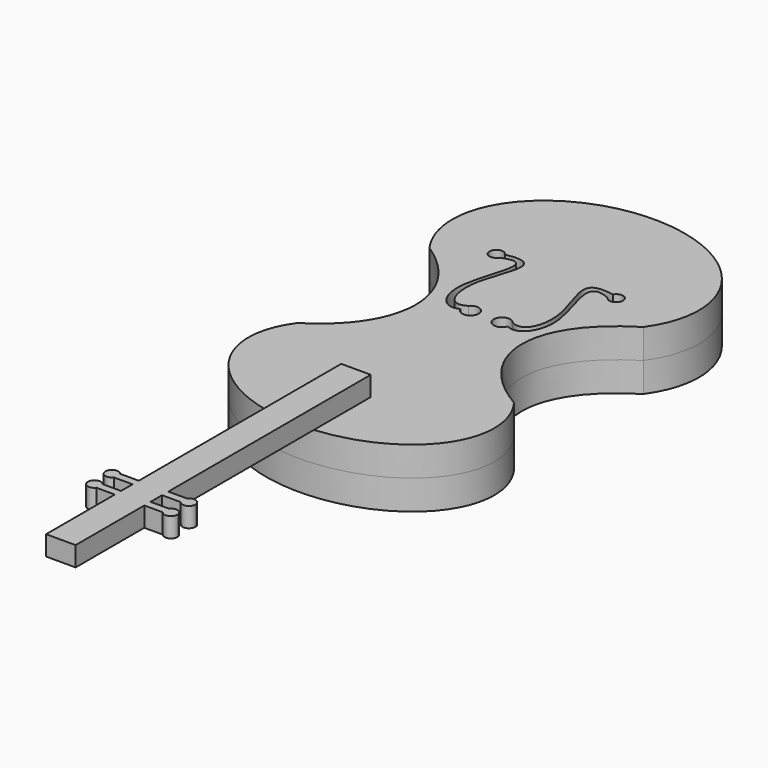
from build123d import *

# Parameters (mm, degrees)
F1_DEPTH = 6
F3_DEPTH = 6
F5_DEPTH = 4
F6_DEPTH = 4


with BuildPart() as f1:
    # F0 (on Top) → F1 (new body)
    with BuildSketch(Plane.XY):
        with BuildLine():
            add(Edge.make_bspline(
                [(-21.7444925397, 18.2306537), (-7.7311441191, 9.1459075591), (-7.7311441191, -6.1719642271), (-21.9778431403, -14.9497014101)],
                knots=[0, 0, 0, 0, 33.1811756533, 33.1811756533, 33.1811756533, 33.1811756533], degree=3))
            add(Edge.make_bspline(
                [(-21.9778431403, -14.9497014101), (-41.9382653472, -42.22478633), (0, -42.22478633), (41.9382653472, -42.22478633), (21.9778431403, -14.9497014101)],
                knots=[2.6455513247, 2.6455513247, 2.6455513247, 4.7123889804, 4.7123889804, 6.779226636, 6.779226636, 6.779226636], degree=2, weights=[1, 0.5118848843, 1, 0.5118848843, 1]))
            add(Edge.make_bspline(
                [(21.7444925397, 18.2306537), (6.4069386012, 8.8349419962), (6.5856454991, -5.9186217795), (21.9778431403, -14.9497014101)],
                knots=[0, 0, 0, 0, 33.1811756533, 33.1811756533, 33.1811756533, 33.1811756533], degree=3))
            add(Edge.make_bspline(
                [(21.7444925397, 18.2306537), (43.2497024841, 48.1910994303), (0, 48.1910994303), (-43.2497024841, 48.1910994303), (-21.7444925397, 18.2306537)],
                knots=[5.7627778356, 5.7627778356, 5.7627778356, 7.853981634, 7.853981634, 9.9451854323, 9.9451854323, 9.9451854323], degree=2, weights=[1, 0.5013812381, 1, 0.5013812381, 1]))
        make_face()
    extrude(amount=F1_DEPTH)

    # F2 (on face) → F3 (join)
    with BuildSketch(Plane.XY.offset(6)):
        with BuildLine():
            add(Edge.make_bspline(
                [(21.7444925397, 18.2306537), (43.2497024841, 48.1910994303), (0, 48.1910994303), (-43.2497024841, 48.1910994303), (-21.7444925397, 18.2306537)],
                knots=[5.7627778356, 5.7627778356, 5.7627778356, 7.853981634, 7.853981634, 9.9451854323, 9.9451854323, 9.9451854323], degree=2, weights=[1, 0.5013812381, 1, 0.5013812381, 1]))
            add(Edge.make_bspline(
                [(-21.7444925397, 18.2306537), (-7.7311441191, 9.1459075591), (-7.7311441191, -6.1719642271), (-21.9778431403, -14.9497014101)],
                knots=[0, 0, 0, 0, 33.1811756533, 33.1811756533, 33.1811756533, 33.1811756533], degree=3))
            add(Edge.make_bspline(
                [(-21.9778431403, -14.9497014101), (-41.9382653472, -42.22478633), (0, -42.22478633), (41.9382653472, -42.22478633), (21.9778431403, -14.9497014101)],
                knots=[2.6455513247, 2.6455513247, 2.6455513247, 4.7123889804, 4.7123889804, 6.779226636, 6.779226636, 6.779226636], degree=2, weights=[1, 0.5118848843, 1, 0.5118848843, 1]))
            add(Edge.make_bspline(
                [(21.7444925397, 18.2306537), (6.4069386012, 8.8349419962), (6.5856454991, -5.9186217795), (21.9778431403, -14.9497014101)],
                knots=[0, 0, 0, 0, 33.1811756533, 33.1811756533, 33.1811756533, 33.1811756533], degree=3))
        make_face()
        with BuildLine():
            add(Edge.make_bspline(
                [(-10.9988739486, 22.5408715923), (-4.1913907555, 25.4376747874), (-13.3990144667, 10.0652438331), (-7.4404065422, 3.5960169038), (-4.885258902, 4.8904192687)],
                knots=[0, 0, 0, 0, 0.5395747944, 1, 1, 1, 1], degree=3))
            ThreePointArc((-10.9988739486, 22.5408715923), (-13.5682932315, 23.2902762166), (-10.9684085473, 23.9259824157))
            add(Edge.make_bspline(
                [(-10.9684085473, 23.9259824157), (-3.068382332, 25.4376747874), (-11.2785667863, 14.0586412607), (-7.7607951045, 4.559221291), (-4.5054177754, 6.5329330973)],
                knots=[0, 0, 0, 0, 0.5227502867, 1, 1, 1, 1], degree=3))
            ThreePointArc((-4.5054177754, 6.5329330973), (-2.6347231367, 7.0482026203), (-1.5180834207, 5.4613450788))
            ThreePointArc((-1.5180834207, 5.4613450788), (-2.9141698346, 3.8005738661), (-4.7901909683, 4.8904192687))
            Line((-4.7901909683, 4.8904192687), (-4.885258902, 4.8904192687))
        make_face(mode=Mode.SUBTRACT)
        with BuildLine():
            ThreePointArc((13.568628233, 23.2598108154), (12.5564550452, 21.9255965626), (10.9988739486, 22.5408715923))
            add(Edge.make_bspline(
                [(10.9988739486, 22.5408715923), (4.1913907555, 25.4376747874), (13.3990144667, 10.0652438331), (7.4404065422, 3.5960169038), (4.885258902, 4.8904192687)],
                knots=[0, 0, 0, 0, 0.5395747944, 1, 1, 1, 1], degree=3))
            Line((4.885258902, 4.8904192687), (4.7901909683, 4.8904192687))
            ThreePointArc((4.7901909683, 4.8904192687), (1.5428641215, 5.1733527098), (4.5054177754, 6.5329330973))
            add(Edge.make_bspline(
                [(10.9684085473, 23.9259824157), (3.068382332, 25.4376747874), (11.2785667863, 14.0586412607), (7.7607951045, 4.559221291), (4.5054177754, 6.5329330973)],
                knots=[0, 0, 0, 0, 0.5227502867, 1, 1, 1, 1], degree=3))
            ThreePointArc((10.9684085473, 23.9259824157), (12.5270259482, 24.6019105709), (13.568628233, 23.2598108154))
        make_face(mode=Mode.SUBTRACT)
    extrude(amount=F3_DEPTH)

    # F4 (on face) → F5 (join)
    with BuildSketch(Plane.XY.offset(12)):
        with BuildLine():
            Line((1.2586822925, -27.6339045167), (0, -27.6339045167))
            Line((0, -27.6339045167), (0, -42.22478633))
            add(Edge.make_bspline(
                [(0, -42.22478633), (1.5054437197, -42.22478633), (3, -42.0911402091)],
                knots=[4.7123889804, 4.7123889804, 4.7123889804, 4.8525318756, 4.8525318756, 4.8525318756], degree=2, weights=[1, 0.966903126, 0.93829455]))
            Line((3, -42.0911402091), (3, -27.6339045167))
            Line((3, -27.6339045167), (1.5, -27.6339045167))
            Line((1.5, -27.6339045167), (1.2586822925, -27.6339045167))
        make_face()
        with BuildLine():
            Line((0, -42.22478633), (0, -27.6339045167))
            Line((0, -27.6339045167), (-1.2586822925, -27.6339045167))
            Line((-1.2586822925, -27.6339045167), (-1.5, -27.6339045167))
            Line((-1.5, -27.6339045167), (-3, -27.6339045167))
            Line((-3, -27.6339045167), (-3, -42.0911402091))
            add(Edge.make_bspline(
                [(-3, -42.0911402091), (-1.5054437197, -42.22478633), (0, -42.22478633)],
                knots=[4.5722460851, 4.5722460851, 4.5722460851, 4.7123889804, 4.7123889804, 4.7123889804], degree=2, weights=[0.93829455, 0.966903126, 1]))
        make_face()
        with BuildLine():
            add(Edge.make_bspline(
                [(0, -42.22478633), (1.5054437197, -42.22478633), (3, -42.0911402091)],
                knots=[4.7123889804, 4.7123889804, 4.7123889804, 4.8525318756, 4.8525318756, 4.8525318756], degree=2, weights=[1, 0.966903126, 0.93829455]))
            Line((0, -42.22478633), (0, -102.6339045167))
            Line((0, -102.6339045167), (3, -102.6339045167))
            Line((3, -102.6339045167), (3, -85.1738639176))
            Line((3, -85.1738639176), (3, -83.5842750967))
            Line((3, -83.5842750967), (3, -80.6650817394))
            Line((3, -80.6650817394), (3, -79.0754929185))
            Line((3, -79.0754929185), (3, -42.0911402091))
        make_face()
        with BuildLine():
            Line((0, -102.6339045167), (0, -42.22478633))
            add(Edge.make_bspline(
                [(-3, -42.0911402091), (-1.5054437197, -42.22478633), (0, -42.22478633)],
                knots=[4.5722460851, 4.5722460851, 4.5722460851, 4.7123889804, 4.7123889804, 4.7123889804], degree=2, weights=[0.93829455, 0.966903126, 1]))
            Line((-3, -42.0911402091), (-3, -79.0754929185))
            Line((-3, -79.0754929185), (-3, -80.6650817394))
            Line((-3, -80.6650817394), (-3, -83.5842750967))
            Line((-3, -83.5842750967), (-3, -85.1738639176))
            Line((-3, -85.1738639176), (-3, -102.6339045167))
            Line((-3, -102.6339045167), (0, -102.6339045167))
        make_face()
    extrude(amount=F5_DEPTH)

    # F4 (on face) → F6 (join)
    with BuildSketch(Plane.XY.offset(12)):
        with BuildLine():
            Line((-6.7470356348, -85.1738639176), (-3, -85.1738639176))
            Line((-3, -85.1738639176), (-3, -83.5842750967))
            Line((-3, -83.5842750967), (-6.7470356348, -83.5842750967))
            ThreePointArc((-6.7470356348, -83.5842750967), (-6.5468067164, -83.9594620601), (-6.477622414, -84.3790695071))
            ThreePointArc((-6.477622414, -84.3790695071), (-6.5468067164, -84.7986769542), (-6.7470356348, -85.1738639176))
        make_face()
        with BuildLine():
            add(Edge.make_bspline(
                [(0, -42.22478633), (1.5054437197, -42.22478633), (3, -42.0911402091)],
                knots=[4.7123889804, 4.7123889804, 4.7123889804, 4.8525318756, 4.8525318756, 4.8525318756], degree=2, weights=[1, 0.966903126, 0.93829455]))
            Line((0, -42.22478633), (0, -102.6339045167))
            Line((0, -102.6339045167), (3, -102.6339045167))
            Line((3, -102.6339045167), (3, -85.1738639176))
            Line((3, -85.1738639176), (3, -83.5842750967))
            Line((3, -83.5842750967), (3, -80.6650817394))
            Line((3, -80.6650817394), (3, -79.0754929185))
            Line((3, -79.0754929185), (3, -42.0911402091))
        make_face()
        with BuildLine():
            Line((7.0841669768, -85.1738639176), (6.7470356348, -85.1738639176))
            ThreePointArc((6.7470356348, -85.1738639176), (8.2042957067, -85.6169510504), (9.0917541053, -84.3790695071))
            ThreePointArc((9.0917541053, -84.3790695071), (8.2042957067, -83.1411879638), (6.7470356348, -83.5842750967))
            Line((6.7470356348, -83.5842750967), (7.0841669768, -83.5842750967))
            Line((7.0841669768, -83.5842750967), (7.0841669768, -85.1738639176))
        make_face()
        with BuildLine():
            Line((6.7970556932, -79.0754929185), (3, -79.0754929185))
            Line((3, -79.0754929185), (3, -80.6650817394))
            Line((3, -80.6650817394), (6.7970556932, -80.6650817394))
            ThreePointArc((6.7970556932, -80.6650817394), (6.5276424725, -79.870287329), (6.7970556932, -79.0754929185))
        make_face()
        with BuildLine():
            ThreePointArc((-6.7470356348, -83.5842750967), (-9.0917541053, -84.3790695071), (-6.7470356348, -85.1738639176))
            Line((-6.7470356348, -85.1738639176), (-7.0841669768, -85.1738639176))
            Line((-7.0841669768, -85.1738639176), (-7.0841669768, -83.5842750967))
            Line((-7.0841669768, -83.5842750967), (-6.7470356348, -83.5842750967))
        make_face()
        with BuildLine():
            Line((0, -42.22478633), (0, -27.6339045167))
            Line((0, -27.6339045167), (-1.2586822925, -27.6339045167))
            Line((-1.2586822925, -27.6339045167), (-1.5, -27.6339045167))
            Line((-1.5, -27.6339045167), (-3, -27.6339045167))
            Line((-3, -27.6339045167), (-3, -42.0911402091))
            add(Edge.make_bspline(
                [(-3, -42.0911402091), (-1.5054437197, -42.22478633), (0, -42.22478633)],
                knots=[4.5722460851, 4.5722460851, 4.5722460851, 4.7123889804, 4.7123889804, 4.7123889804], degree=2, weights=[0.93829455, 0.966903126, 1]))
        make_face()
        with BuildLine():
            Line((3, -83.5842750967), (3, -85.1738639176))
            Line((3, -85.1738639176), (6.7470356348, -85.1738639176))
            ThreePointArc((6.7470356348, -85.1738639176), (6.477622414, -84.3790695071), (6.7470356348, -83.5842750967))
            Line((6.7470356348, -83.5842750967), (3, -83.5842750967))
        make_face()
        with BuildLine():
            Line((-7.1341870353, -79.0754929185), (-6.7970556932, -79.0754929185))
            ThreePointArc((-6.7970556932, -79.0754929185), (-9.1417741638, -79.870287329), (-6.7970556932, -80.6650817394))
            Line((-6.7970556932, -80.6650817394), (-7.1341870353, -80.6650817394))
            Line((-7.1341870353, -80.6650817394), (-7.1341870353, -79.0754929185))
        make_face()
        with BuildLine():
            Line((7.1341870353, -79.0754929185), (6.7970556932, -79.0754929185))
            ThreePointArc((6.7970556932, -79.0754929185), (6.5276424725, -79.870287329), (6.7970556932, -80.6650817394))
            Line((6.7970556932, -80.6650817394), (7.1341870353, -80.6650817394))
            Line((7.1341870353, -80.6650817394), (7.1341870353, -79.0754929185))
        make_face()
        with BuildLine():
            ThreePointArc((-6.5276424725, -79.870287329), (-6.5968267748, -79.4506798819), (-6.7970556932, -79.0754929185))
            Line((-6.7970556932, -79.0754929185), (-7.1341870353, -79.0754929185))
            Line((-7.1341870353, -79.0754929185), (-7.1341870353, -80.6650817394))
            Line((-7.1341870353, -80.6650817394), (-6.7970556932, -80.6650817394))
            ThreePointArc((-6.7970556932, -80.6650817394), (-6.5968267748, -80.289894776), (-6.5276424725, -79.870287329))
        make_face()
        with BuildLine():
            ThreePointArc((6.7470356348, -83.5842750967), (6.477622414, -84.3790695071), (6.7470356348, -85.1738639176))
            Line((6.7470356348, -85.1738639176), (7.0841669768, -85.1738639176))
            Line((7.0841669768, -85.1738639176), (7.0841669768, -83.5842750967))
            Line((7.0841669768, -83.5842750967), (6.7470356348, -83.5842750967))
        make_face()
        with BuildLine():
            Line((-7.0841669768, -85.1738639176), (-6.7470356348, -85.1738639176))
            ThreePointArc((-6.7470356348, -85.1738639176), (-6.5468067164, -84.7986769542), (-6.477622414, -84.3790695071))
            ThreePointArc((-6.477622414, -84.3790695071), (-6.5468067164, -83.9594620601), (-6.7470356348, -83.5842750967))
            Line((-6.7470356348, -83.5842750967), (-7.0841669768, -83.5842750967))
            Line((-7.0841669768, -83.5842750967), (-7.0841669768, -85.1738639176))
        make_face()
        with BuildLine():
            Line((-3, -80.6650817394), (-3, -79.0754929185))
            Line((-3, -79.0754929185), (-6.7970556932, -79.0754929185))
            ThreePointArc((-6.7970556932, -79.0754929185), (-6.5968267748, -79.4506798819), (-6.5276424725, -79.870287329))
            ThreePointArc((-6.5276424725, -79.870287329), (-6.5968267748, -80.289894776), (-6.7970556932, -80.6650817394))
            Line((-6.7970556932, -80.6650817394), (-3, -80.6650817394))
        make_face()
        with BuildLine():
            Line((0, -102.6339045167), (0, -42.22478633))
            add(Edge.make_bspline(
                [(-3, -42.0911402091), (-1.5054437197, -42.22478633), (0, -42.22478633)],
                knots=[4.5722460851, 4.5722460851, 4.5722460851, 4.7123889804, 4.7123889804, 4.7123889804], degree=2, weights=[0.93829455, 0.966903126, 1]))
            Line((-3, -42.0911402091), (-3, -79.0754929185))
            Line((-3, -79.0754929185), (-3, -80.6650817394))
            Line((-3, -80.6650817394), (-3, -83.5842750967))
            Line((-3, -83.5842750967), (-3, -85.1738639176))
            Line((-3, -85.1738639176), (-3, -102.6339045167))
            Line((-3, -102.6339045167), (0, -102.6339045167))
        make_face()
        with BuildLine():
            ThreePointArc((9.1417741638, -79.870287329), (8.2543157651, -78.6324057857), (6.7970556932, -79.0754929185))
            Line((6.7970556932, -79.0754929185), (7.1341870353, -79.0754929185))
            Line((7.1341870353, -79.0754929185), (7.1341870353, -80.6650817394))
            Line((7.1341870353, -80.6650817394), (6.7970556932, -80.6650817394))
            ThreePointArc((6.7970556932, -80.6650817394), (8.2543157651, -81.1081688723), (9.1417741638, -79.870287329))
        make_face()
    extrude(amount=F6_DEPTH)


solid = f1.part
